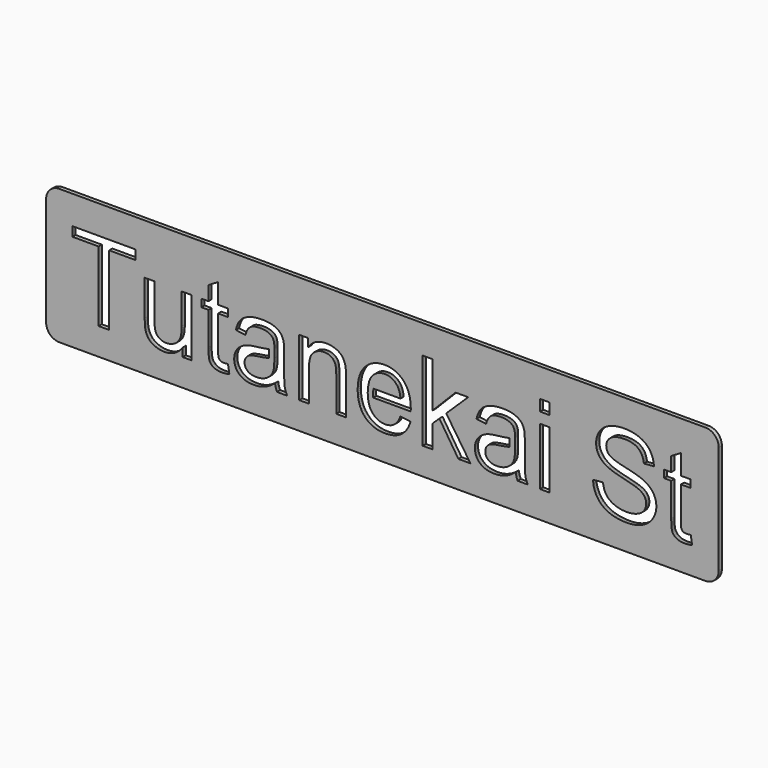
from build123d import *

# Parameters (mm, degrees)
F0_W     = 7.366985
F0_H     = 43.465212
F0_H_2   = 8.472032
F1_DEPTH = 3


# Not quite as in the source:
# - ends of sketch curves that miss each other by under 0.0002 mm in the source are joined


with BuildPart() as f1:
    # F0 (on Front) → F1 (new body)
    with BuildSketch(Plane.XZ):
        with BuildLine():
            Line((-254, 41), (-254, -41))
            ThreePointArc((-254, -41), (-251.0710678119, -48.0710678119), (-244, -51))
            Line((-244, -51), (244, -51))
            ThreePointArc((244, -51), (251.0710678119, -48.0710678119), (254, -41))
            Line((254, -41), (254, 41))
            ThreePointArc((254, 41), (251.0710678119, 48.0710678119), (244, 51))
            Line((244, 51), (-244, 51))
            ThreePointArc((-244, 51), (-251.0710678119, 48.0710678119), (-254, 41))
        make_face()
        Polygon((-206.388994, 22.359541), (-206.388994, -30.559968), (-214.328967, -30.559968), (-214.328967, 22.359541), (-234.097043, 22.359541), (-234.097043, 29.440032), (-186.539063, 29.440032), (-186.539063, 22.359541), align=None, mode=Mode.SUBTRACT)
        Polygon((-144.260754, 12.905244), (-144.260754, -30.559968), (-150.850113, -30.559968), (-150.850113, -24.175247), (-151.498721, -25.067343), (-152.175787, -25.901884), (-152.88131, -26.678871), (-153.61529, -27.398303), (-154.377729, -28.060181), (-155.168624, -28.664504), (-155.987977, -29.211272), (-156.835788, -29.700486), (-157.712057, -30.132145), (-158.616782, -30.50625), (-159.549966, -30.8228), (-160.511607, -31.081796), (-161.501705, -31.283237), (-162.520261, -31.427123), (-163.567275, -31.513455), (-164.642746, -31.542232), (-165.596553, -31.51921), (-166.534373, -31.450145), (-167.456205, -31.335036), (-168.36205, -31.173883), (-169.251908, -30.966686), (-170.125778, -30.713446), (-170.983661, -30.414163), (-171.825556, -30.068835), (-172.632599, -29.688655), (-173.385925, -29.284814), (-174.085532, -28.857311), (-174.731423, -28.406148), (-175.323595, -27.931322), (-175.86205, -27.432836), (-176.346788, -26.910688), (-176.777807, -26.364879), (-177.16694, -25.791571), (-177.526017, -25.186929), (-177.855037, -24.550951), (-178.154001, -23.883637), (-178.422909, -23.184989), (-178.66176, -22.455005), (-178.870556, -21.693686), (-179.049294, -20.901032), (-179.154811, -20.319091), (-179.246259, -19.657853), (-179.323638, -18.917317), (-179.386948, -18.097485), (-179.436189, -17.198354), (-179.471361, -16.219927), (-179.492465, -15.162201), (-179.499499, -14.025179), (-179.499499, 12.905244), (-172.132514, 12.905244), (-172.132514, -11.201168), (-172.130755, -11.90781), (-172.12548, -12.585036), (-172.116687, -13.232844), (-172.104376, -13.851236), (-172.088549, -14.440211), (-172.069204, -14.99977), (-172.046342, -15.529911), (-172.019963, -16.030636), (-171.990067, -16.501944), (-171.956653, -16.943835), (-171.919722, -17.35631), (-171.879274, -17.739367), (-171.835309, -18.093008), (-171.787826, -18.417232), (-171.736826, -18.712039), (-171.682309, -18.97743), (-171.484066, -19.684392), (-171.237221, -20.352345), (-170.941774, -20.981288), (-170.597726, -21.571223), (-170.205075, -22.122148), (-169.763824, -22.634064), (-169.27397, -23.10697), (-168.735515, -23.540868), (-168.156133, -23.929361), (-167.543496, -24.266056), (-166.897606, -24.550951), (-166.218462, -24.784047), (-165.506065, -24.965344), (-164.760413, -25.094841), (-163.981508, -25.17254), (-163.169349, -25.19844), (-162.346958, -25.171901), (-161.537357, -25.092283), (-160.740546, -24.959588), (-159.956525, -24.773815), (-159.185294, -24.534963), (-158.426852, -24.243034), (-157.681201, -23.898026), (-156.948339, -23.49994), (-156.248412, -23.056131), (-155.601563, -22.573951), (-155.007791, -22.053402), (-154.467098, -21.494483), (-153.979483, -20.897195), (-153.544946, -20.261536), (-153.163487, -19.587508), (-152.835106, -18.875111), (-152.55213, -18.102281), (-152.306883, -17.246956), (-152.099367, -16.309136), (-151.929581, -15.288822), (-151.797525, -14.186012), (-151.7032, -13.000708), (-151.646604, -11.732908), (-151.627739, -10.382614), (-151.627739, 12.905244), align=None, mode=Mode.SUBTRACT)
        Polygon((-97.552982, 7.077844), (-97.979446, 6.928442), (-98.384646, 6.764811), (-98.768583, 6.586951), (-99.131256, 6.394863), (-99.472667, 6.188546), (-99.792814, 5.968), (-100.097294, 5.729388), (-100.391701, 5.468874), (-100.676037, 5.186457), (-100.950301, 4.882137), (-101.214492, 4.555914), (-101.468611, 4.207789), (-101.712659, 3.837761), (-101.946634, 3.445831), (-102.170537, 3.031997), (-102.384369, 2.596261), (-102.588128, 2.138622), (-102.781815, 1.659081), (-102.96543, 1.157637), (-103.138973, 0.63429), (-103.302444, 0.08904), (-103.455843, -0.478112), (-110.659117, 0.504153), (-110.393727, 1.632542), (-110.088687, 2.705295), (-109.743999, 3.722412), (-109.359663, 4.683893), (-108.935677, 5.589738), (-108.472043, 6.439947), (-107.968761, 7.23452), (-107.425829, 7.973457), (-106.831738, 8.664112), (-106.174977, 9.313839), (-105.455544, 9.922638), (-104.673442, 10.49051), (-103.828669, 11.017454), (-102.921225, 11.50347), (-101.951111, 11.948559), (-100.918326, 12.35272), (-99.833102, 12.712436), (-98.705672, 13.02419), (-97.536036, 13.287982), (-96.324192, 13.503811), (-95.070142, 13.671679), (-93.773885, 13.791584), (-92.435422, 13.863528), (-91.054751, 13.887509), (-89.695824, 13.867045), (-88.402125, 13.805653), (-87.173655, 13.703334), (-86.010413, 13.560087), (-84.9124, 13.375912), (-83.879615, 13.15081), (-82.912059, 12.88478), (-82.009731, 12.577822), (-81.168795, 12.239849), (-80.385413, 11.880773), (-79.659586, 11.500593), (-78.991314, 11.099309), (-78.380596, 10.676923), (-77.827432, 10.233433), (-77.331823, 9.76884), (-76.893769, 9.283143), (-76.49984, 8.770588), (-76.136607, 8.225418), (-75.804069, 7.647634), (-75.502228, 7.037236), (-75.231082, 6.394223), (-74.990631, 5.718597), (-74.780877, 5.010356), (-74.601818, 4.2695), (-74.515486, 3.751509), (-74.440666, 3.138873), (-74.377355, 2.431591), (-74.325556, 1.629664), (-74.285268, 0.733092), (-74.256491, -0.258126), (-74.239225, -1.343989), (-74.233469, -2.524497), (-74.233469, -12.347144), (-74.231631, -13.601753), (-74.226115, -14.797369), (-74.216922, -15.933992), (-74.204052, -17.011622), (-74.187505, -18.030258), (-74.167281, -18.9899), (-74.14338, -19.890549), (-74.115802, -20.732205), (-74.084547, -21.514867), (-74.049614, -22.238536), (-74.011005, -22.903211), (-73.968718, -23.508893), (-73.922754, -24.055582), (-73.873113, -24.543277), (-73.819796, -24.971978), (-73.762801, -25.341686), (-73.630745, -26.018592), (-73.469912, -26.688463), (-73.280301, -27.3513), (-73.061914, -28.007103), (-72.814749, -28.65587), (-72.538807, -29.297604), (-72.234087, -29.932303), (-71.90059, -30.559968), (-79.594997, -30.559968), (-79.868701, -29.974829), (-80.116825, -29.36539), (-80.339369, -28.731651), (-80.536334, -28.07361), (-80.707719, -27.391269), (-80.853524, -26.684626), (-80.973749, -25.953683), (-81.068394, -25.19844), (-82.08679, -26.036178), (-83.095594, -26.809968), (-84.094805, -27.519807), (-85.084424, -28.165697), (-86.06445, -28.747638), (-87.034884, -29.265629), (-87.995726, -29.719671), (-88.946975, -30.109763), (-89.902061, -30.445498), (-90.874414, -30.736468), (-91.864033, -30.982674), (-92.870918, -31.184115), (-93.895069, -31.340791), (-94.936487, -31.452703), (-95.995172, -31.51985), (-97.071123, -31.542232), (-97.953466, -31.528563), (-98.80991, -31.487555), (-99.640454, -31.419209), (-100.445099, -31.323525), (-101.223845, -31.200502), (-101.97669, -31.050141), (-102.703637, -30.872441), (-103.404683, -30.667403), (-104.07983, -30.435026), (-104.729078, -30.175311), (-105.352426, -29.888258), (-105.949874, -29.573866), (-106.521423, -29.232136), (-107.067072, -28.863067), (-107.586822, -28.46666), (-108.080672, -28.042914), (-108.546545, -27.597906), (-108.982361, -27.137709), (-109.38812, -26.662324), (-109.763824, -26.171751), (-110.109471, -25.665991), (-110.425062, -25.145042), (-110.710596, -24.608905), (-110.966075, -24.05758), (-111.191497, -23.491067), (-111.386863, -22.909366), (-111.552172, -22.312478), (-111.687425, -21.700401), (-111.792622, -21.073136), (-111.867763, -20.430683), (-111.912847, -19.773042), (-111.927876, -19.100213), (-111.905174, -18.310756), (-111.837067, -17.538566), (-111.723557, -16.783642), (-111.564642, -16.045984), (-111.360324, -15.325593), (-111.110601, -14.622468), (-110.815474, -13.936609), (-110.474942, -13.268017), (-110.09764, -12.624365), (-109.6922, -12.013327), (-109.258623, -11.434904), (-108.796907, -10.889094), (-108.307054, -10.375899), (-107.789063, -9.895319), (-107.242934, -9.447352), (-106.668667, -9.032), (-106.071059, -8.645106), (-105.454905, -8.282512), (-104.820206, -7.944219), (-104.166962, -7.630227), (-103.495172, -7.340535), (-102.804837, -7.075145), (-102.095956, -6.834055), (-101.36853, -6.617266), (-100.791706, -6.474659), (-100.145816, -6.33333), (-99.43086, -6.193281), (-98.646839, -6.05451), (-97.793752, -5.917019), (-96.8716, -5.780807), (-95.880382, -5.645873), (-94.820099, -5.512219), (-93.723205, -5.377605), (-92.663082, -5.239794), (-91.63973, -5.098785), (-90.653148, -4.954579), (-89.703338, -4.807175), (-88.790299, -4.656574), (-87.914031, -4.502775), (-87.074533, -4.345779), (-86.271807, -4.185586), (-85.674982, -4.058273), (-85.684298, -10.013809), (-85.959573, -10.08397), (-86.695952, -10.259831), (-87.463666, -10.431855), (-88.262715, -10.600043), (-89.0931, -10.764393), (-89.95482, -10.924906), (-90.847875, -11.081582), (-91.772265, -11.234422), (-92.727991, -11.383424), (-93.715052, -11.52859), (-94.809228, -11.694858), (-95.82027, -11.866243), (-96.748177, -12.042744), (-97.592951, -12.22436), (-98.354589, -12.411093), (-99.033094, -12.602942), (-99.628464, -12.799906), (-100.1407, -13.001987), (-100.597939, -13.218456), (-101.028319, -13.458586), (-101.43184, -13.722378), (-101.808503, -14.009831), (-102.158307, -14.320946), (-102.481252, -14.655721), (-102.777338, -15.014158), (-103.046566, -15.396257), (-103.286377, -15.795622), (-103.494213, -16.205858), (-103.670074, -16.626965), (-103.81396, -17.058944), (-103.925872, -17.501795), (-104.005809, -17.955517), (-104.053771, -18.42011), (-104.069758, -18.895575), (-104.034906, -19.616925), (-103.930348, -20.30758), (-103.756086, -20.967539), (-103.512118, -21.596802), (-103.198446, -22.19537), (-102.815069, -22.763242), (-102.361986, -23.300418), (-101.839199, -23.806898), (-101.249265, -24.267335), (-100.594741, -24.66638), (-99.875629, -25.004033), (-99.091927, -25.280295), (-98.243637, -25.495165), (-97.330758, -25.648644), (-96.353289, -25.740732), (-95.311232, -25.771427), (-94.26182, -25.74233), (-93.241825, -25.655039), (-92.251247, -25.509554), (-91.290086, -25.305875), (-90.358341, -25.044001), (-89.456013, -24.723934), (-88.583102, -24.345673), (-87.739608, -23.909217), (-86.938321, -23.422242), (-86.19203, -22.89242), (-85.500735, -22.319752), (-84.864438, -21.704238), (-84.283137, -21.045877), (-83.756832, -20.344671), (-83.285524, -19.600618), (-82.869213, -18.813719), (-82.591032, -18.152481), (-82.349942, -17.417062), (-82.145943, -16.607461), (-81.979035, -15.723678), (-81.849218, -14.765714), (-81.756491, -13.733569), (-81.700855, -12.627242), (-81.682309, -11.446734), (-81.682309, -8.745506), (-81.672717, -2.613387), (-81.664404, -2.286605), (-81.657369, -1.994355), (-81.651614, -1.736639), (-81.647137, -1.513455), (-81.64394, -1.324804), (-81.642021, -1.170685), (-81.641382, -1.0511), (-81.649535, -0.498736), (-81.673996, 0.032845), (-81.714764, 0.543641), (-81.771839, 1.033655), (-81.845221, 1.502884), (-81.93491, 1.95133), (-82.040906, 2.378993), (-82.16321, 2.785871), (-82.30182, 3.171967), (-82.456738, 3.537278), (-82.627963, 3.881806), (-82.815495, 4.205551), (-83.019334, 4.508512), (-83.23948, 4.790689), (-83.475934, 5.052083), (-83.728694, 5.292693), (-84.092407, 5.595014), (-84.477543, 5.877831), (-84.884102, 6.141143), (-85.312084, 6.384951), (-85.76149, 6.609254), (-86.232318, 6.814052), (-86.724569, 6.999346), (-87.238244, 7.165135), (-87.773342, 7.311419), (-88.329862, 7.438199), (-88.907806, 7.545475), (-89.507173, 7.633245), (-90.127963, 7.701511), (-90.770176, 7.750273), (-91.433812, 7.77953), (-92.118872, 7.789282), (-92.757967, 7.782168), (-93.375799, 7.760825), (-93.972368, 7.725253), (-94.547674, 7.675452), (-95.101717, 7.611423), (-95.634497, 7.533164), (-96.146013, 7.440677), (-96.636266, 7.333962), (-97.105256, 7.213017), align=None, mode=Mode.SUBTRACT)
        Polygon((-117.588687, -24.09595), (-117.123774, -24.037756), (-116.63456, -23.970609), (-115.57044, -30.478112), (-116.337835, -30.631591), (-117.084765, -30.764606), (-117.811232, -30.877157), (-118.517234, -30.969244), (-119.202773, -31.040868), (-119.867848, -31.092028), (-120.51246, -31.122723), (-121.136607, -31.132955), (-122.111198, -31.113131), (-123.029513, -31.053658), (-123.891552, -30.954536), (-124.697316, -30.815766), (-125.446805, -30.637346), (-126.140017, -30.419279), (-126.776955, -30.161562), (-127.357616, -29.864197), (-127.889676, -29.534537), (-128.380809, -29.179937), (-128.831013, -28.800396), (-129.24029, -28.395916), (-129.60864, -27.966495), (-129.936061, -27.512133), (-130.222555, -27.032832), (-130.468121, -26.52859), (-130.577155, -26.252408), (-130.679155, -25.940574), (-130.77412, -25.593088), (-130.86205, -25.20995), (-130.942946, -24.791161), (-131.016808, -24.33672), (-131.083635, -23.846627), (-131.143428, -23.320882), (-131.196186, -22.759485), (-131.24191, -22.162436), (-131.2806, -21.529735), (-131.312255, -20.861383), (-131.336875, -20.157379), (-131.354462, -19.417722), (-131.365013, -18.642414), (-131.36853, -17.831455), (-131.36853, 7.175367), (-136.770986, 7.175367), (-136.770986, 12.905244), (-131.36853, 12.905244), (-131.36853, 23.669228), (-124.042473, 28.089419), (-124.042473, 12.905244), (-116.63456, 12.905244), (-116.63456, 7.175367), (-124.042473, 7.175367), (-124.042473, -18.240732), (-124.036398, -18.993417), (-124.018172, -19.675759), (-123.987796, -20.287756), (-123.94527, -20.829408), (-123.890593, -21.300716), (-123.823766, -21.70168), (-123.744788, -22.032299), (-123.65366, -22.292573), (-123.428558, -22.719756), (-123.142064, -23.100895), (-122.794178, -23.435991), (-122.384902, -23.725043), (-122.153085, -23.849744), (-121.897606, -23.957819), (-121.618466, -24.049267), (-121.315666, -24.124088), (-120.989203, -24.182282), (-120.63908, -24.223849), (-120.265295, -24.248789), (-119.867848, -24.257103), (-119.54874, -24.252626), (-119.205331, -24.239197), (-118.837622, -24.216814), (-118.445611, -24.185479), (-118.0293, -24.145191), align=None, mode=Mode.SUBTRACT)
        Polygon((-55.447657, -6.821905), (-55.447657, -30.559968), (-62.814642, -30.559968), (-62.814642, 12.905244), (-56.184356, 12.905244), (-56.184356, 6.725162), (-55.569161, 7.592477), (-54.920713, 8.403837), (-54.239011, 9.159241), (-53.524056, 9.858689), (-52.775846, 10.502181), (-51.994383, 11.089717), (-51.179666, 11.621297), (-50.331696, 12.096922), (-49.450471, 12.516591), (-48.535993, 12.880304), (-47.588261, 13.188061), (-46.607275, 13.439862), (-45.593036, 13.635707), (-44.545543, 13.775597), (-43.464796, 13.859531), (-42.350795, 13.887509), (-41.378443, 13.865446), (-40.425914, 13.799258), (-39.493211, 13.688945), (-38.580331, 13.534507), (-37.687276, 13.335944), (-36.814045, 13.093256), (-35.960639, 12.806442), (-35.127057, 12.475503), (-34.329287, 12.108753), (-33.583316, 11.714504), (-32.889144, 11.292757), (-32.246771, 10.843511), (-31.656197, 10.366768), (-31.117422, 9.862526), (-30.630446, 9.330785), (-30.19527, 8.771547), (-29.801341, 8.18513), (-29.438108, 7.571854), (-29.10557, 6.931719), (-28.803728, 6.264726), (-28.532582, 5.570873), (-28.292132, 4.850162), (-28.082378, 4.102592), (-27.903319, 3.328163), (-27.853758, 3.060375), (-27.807395, 2.768605), (-27.764229, 2.452854), (-27.72426, 2.113123), (-27.687489, 1.74941), (-27.653916, 1.361716), (-27.62354, 0.950041), (-27.596361, 0.514384), (-27.57238, 0.054747), (-27.551597, -0.428871), (-27.53401, -0.93647), (-27.519622, -1.468051), (-27.508431, -2.023612), (-27.500437, -2.603155), (-27.495641, -3.206678), (-27.494042, -3.834183), (-27.494042, -30.559968), (-34.861027, -30.559968), (-34.861027, -4.120677), (-34.874456, -3.030657), (-34.914745, -2.011622), (-34.981892, -1.06357), (-35.075897, -0.186502), (-35.196762, 0.619581), (-35.344485, 1.354681), (-35.519068, 2.018797), (-35.720509, 2.611929), (-35.956163, 3.1555), (-36.233384, 3.670933), (-36.552172, 4.158228), (-36.912528, 4.617386), (-37.31445, 5.048406), (-37.75794, 5.451288), (-38.242998, 5.826032), (-38.769622, 6.172638), (-39.32886, 6.484392), (-39.91176, 6.754579), (-40.518322, 6.983198), (-41.148544, 7.170251), (-41.802428, 7.315736), (-42.479973, 7.419654), (-43.18118, 7.482005), (-43.906047, 7.502788), (-44.489347, 7.491117), (-45.062575, 7.456105), (-45.62573, 7.397751), (-46.178814, 7.316056), (-46.721825, 7.211019), (-47.254764, 7.08264), (-47.777632, 6.93092), (-48.290427, 6.755858), (-48.79315, 6.557454), (-49.285801, 6.335709), (-49.76838, 6.090623), (-50.240887, 5.822195), (-50.703322, 5.530425), (-51.155685, 5.215314), (-51.597976, 4.876861), (-52.030195, 4.515067), (-52.444028, 4.120658), (-52.831163, 3.684362), (-53.191598, 3.20618), (-53.525335, 2.68611), (-53.832372, 2.124154), (-54.112711, 1.52031), (-54.366351, 0.87458), (-54.593292, 0.186963), (-54.793534, -0.542541), (-54.967077, -1.313932), (-55.113921, -2.12721), (-55.234066, -2.982375), (-55.327512, -3.879427), (-55.394259, -4.818366), (-55.434308, -5.799192), align=None, mode=Mode.SUBTRACT)
        with BuildLine():
            Line((-5.055434, -23.343903), (-4.536803, -23.685873))
            Line((-4.536803, -23.685873), (-4.004103, -23.998107))
            Line((-4.004103, -23.998107), (-3.457335, -24.280604))
            Line((-3.457335, -24.280604), (-2.896498, -24.533365))
            Line((-2.896498, -24.533365), (-2.321591, -24.756388))
            Line((-2.321591, -24.756388), (-1.732616, -24.949676))
            Line((-1.732616, -24.949676), (-1.129572, -25.113227))
            Line((-1.129572, -25.113227), (-0.51246, -25.247041))
            Line((-0.51246, -25.247041), (0.118722, -25.351119))
            Line((0.118722, -25.351119), (0.763973, -25.42546))
            Line((0.763973, -25.42546), (1.423293, -25.470065))
            Line((1.423293, -25.470065), (2.096681, -25.484933))
            Line((2.096681, -25.484933), (3.091096, -25.45168))
            Line((3.091096, -25.45168), (4.04842, -25.351918))
            Line((4.04842, -25.351918), (4.968654, -25.18565))
            Line((4.968654, -25.18565), (5.851797, -24.952873))
            Line((5.851797, -24.952873), (6.697849, -24.65359))
            Line((6.697849, -24.65359), (7.506811, -24.287798))
            Line((7.506811, -24.287798), (8.278681, -23.8555))
            Line((8.278681, -23.8555), (9.013461, -23.356693))
            Line((9.013461, -23.356693), (9.711151, -22.784985))
            Line((9.711151, -22.784985), (10.371749, -22.133978))
            Line((10.371749, -22.133978), (10.995257, -21.403675))
            Line((10.995257, -21.403675), (11.581674, -20.594074))
            Line((11.581674, -20.594074), (12.131001, -19.705176))
            Line((12.131001, -19.705176), (12.643236, -18.73698))
            Line((12.643236, -18.73698), (13.118381, -17.689487))
            Line((13.118381, -17.689487), (13.556435, -16.562696))
            Line((13.556435, -16.562696), (21.168987, -17.504033))
            Line((21.168987, -17.504033), (20.931894, -18.326264))
            Line((20.931894, -18.326264), (20.67082, -19.125153))
            Line((20.67082, -19.125153), (20.385765, -19.900701))
            Line((20.385765, -19.900701), (20.076729, -20.652907))
            Line((20.076729, -20.652907), (19.743712, -21.381772))
            Line((19.743712, -21.381772), (19.386713, -22.087295))
            Line((19.386713, -22.087295), (19.005734, -22.769477))
            Line((19.005734, -22.769477), (18.600774, -23.428317))
            Line((18.600774, -23.428317), (18.171832, -24.063815))
            Line((18.171832, -24.063815), (17.71891, -24.675972))
            Line((17.71891, -24.675972), (17.242006, -25.264787))
            Line((17.242006, -25.264787), (16.741122, -25.830261))
            Line((16.741122, -25.830261), (16.216256, -26.372393))
            Line((16.216256, -26.372393), (15.667409, -26.891183))
            Line((15.667409, -26.891183), (15.094581, -27.386632))
            Line((15.094581, -27.386632), (14.497772, -27.85874))
            Line((14.497772, -27.85874), (13.878421, -28.304788))
            Line((13.878421, -28.304788), (13.237967, -28.722058))
            Line((13.237967, -28.722058), (12.576409, -29.110552))
            Line((12.576409, -29.110552), (11.893748, -29.470268))
            Line((11.893748, -29.470268), (11.189983, -29.801206))
            Line((11.189983, -29.801206), (10.465116, -30.103368))
            Line((10.465116, -30.103368), (9.719144, -30.376752))
            Line((9.719144, -30.376752), (8.95207, -30.621359))
            Line((8.95207, -30.621359), (8.163892, -30.837189))
            Line((8.163892, -30.837189), (7.354611, -31.024241))
            Line((7.354611, -31.024241), (6.524226, -31.182516))
            Line((6.524226, -31.182516), (5.672738, -31.312014))
            Line((5.672738, -31.312014), (4.800147, -31.412734))
            Line((4.800147, -31.412734), (3.906453, -31.484678))
            Line((3.906453, -31.484678), (2.991655, -31.527844))
            Line((2.991655, -31.527844), (2.055753, -31.542232))
            Line((2.055753, -31.542232), (0.879162, -31.51929))
            Line((0.879162, -31.51929), (-0.266574, -31.450465))
            Line((-0.266574, -31.450465), (-1.381454, -31.335755))
            Line((-1.381454, -31.335755), (-2.465478, -31.175162))
            Line((-2.465478, -31.175162), (-3.518647, -30.968685))
            Line((-3.518647, -30.968685), (-4.54096, -30.716324))
            Line((-4.54096, -30.716324), (-5.532417, -30.41808))
            Line((-5.532417, -30.41808), (-6.493019, -30.073951))
            Line((-6.493019, -30.073951), (-7.422765, -29.683939))
            Line((-7.422765, -29.683939), (-8.321655, -29.248043))
            Line((-8.321655, -29.248043), (-9.18969, -28.766263))
            Line((-9.18969, -28.766263), (-10.026869, -28.2386))
            Line((-10.026869, -28.2386), (-10.833193, -27.665053))
            Line((-10.833193, -27.665053), (-11.608661, -27.045622))
            Line((-11.608661, -27.045622), (-12.353273, -26.380307))
            Line((-12.353273, -26.380307), (-13.06703, -25.669108))
            Line((-13.06703, -25.669108), (-13.743536, -24.916502))
            Line((-13.743536, -24.916502), (-14.376396, -24.126965))
            Line((-14.376396, -24.126965), (-14.965611, -23.300498))
            Line((-14.965611, -23.300498), (-15.511181, -22.437099))
            Line((-15.511181, -22.437099), (-16.013104, -21.53677))
            Line((-16.013104, -21.53677), (-16.471383, -20.59951))
            Line((-16.471383, -20.59951), (-16.886015, -19.625319))
            Line((-16.886015, -19.625319), (-17.257002, -18.614197))
            Line((-17.257002, -18.614197), (-17.584344, -17.566144))
            Line((-17.584344, -17.566144), (-17.86804, -16.48116))
            Line((-17.86804, -16.48116), (-18.108091, -15.359246))
            Line((-18.108091, -15.359246), (-18.304496, -14.200401))
            Line((-18.304496, -14.200401), (-18.457255, -13.004625))
            Line((-18.457255, -13.004625), (-18.566369, -11.771918))
            Line((-18.566369, -11.771918), (-18.631837, -10.50228))
            Line((-18.631837, -10.50228), (-18.65366, -9.195711))
            Line((-18.65366, -9.195711), (-18.631597, -7.843818))
            Line((-18.631597, -7.843818), (-18.56541, -6.530295))
            Line((-18.56541, -6.530295), (-18.455097, -5.255141))
            Line((-18.455097, -5.255141), (-18.300659, -4.018358))
            Line((-18.300659, -4.018358), (-18.102095, -2.819944))
            Line((-18.102095, -2.819944), (-17.859407, -1.659899))
            Line((-17.859407, -1.659899), (-17.572593, -0.538225))
            Line((-17.572593, -0.538225), (-17.241655, 0.54508))
            Line((-17.241655, 0.54508), (-16.866591, 1.590015))
            Line((-16.866591, 1.590015), (-16.447402, 2.596581))
            Line((-16.447402, 2.596581), (-15.984087, 3.564777))
            Line((-15.984087, 3.564777), (-15.476648, 4.494603))
            Line((-15.476648, 4.494603), (-14.925083, 5.386059))
            Line((-14.925083, 5.386059), (-14.329393, 6.239146))
            Line((-14.329393, 6.239146), (-13.689578, 7.053863))
            Line((-13.689578, 7.053863), (-13.005638, 7.83021))
            Line((-13.005638, 7.83021), (-12.286526, 8.563711))
            Line((-12.286526, 8.563711), (-11.541194, 9.249889))
            Line((-11.541194, 9.249889), (-10.769643, 9.888745))
            Line((-10.769643, 9.888745), (-9.971873, 10.480278))
            Line((-9.971873, 10.480278), (-9.147883, 11.024488))
            Line((-9.147883, 11.024488), (-8.297674, 11.521376))
            Line((-8.297674, 11.521376), (-7.421246, 11.970941))
            Line((-7.421246, 11.970941), (-6.518599, 12.373184))
            Line((-6.518599, 12.373184), (-5.589732, 12.728104))
            Line((-5.589732, 12.728104), (-4.634646, 13.035701))
            Line((-4.634646, 13.035701), (-3.65334, 13.295976))
            Line((-3.65334, 13.295976), (-2.645816, 13.508927))
            Line((-2.645816, 13.508927), (-1.612072, 13.674557))
            Line((-1.612072, 13.674557), (-0.552108, 13.792863))
            Line((-0.552108, 13.792863), (0.534074, 13.863847))
            Line((0.534074, 13.863847), (1.646476, 13.887509))
            Line((1.646476, 13.887509), (2.723706, 13.864327))
            Line((2.723706, 13.864327), (3.775995, 13.794782))
            Line((3.775995, 13.794782), (4.803345, 13.678873))
            Line((4.803345, 13.678873), (5.805753, 13.516601))
            Line((5.805753, 13.516601), (6.783222, 13.307966))
            Line((6.783222, 13.307966), (7.73575, 13.052967))
            Line((7.73575, 13.052967), (8.663338, 12.751605))
            Line((8.663338, 12.751605), (9.565985, 12.40388))
            Line((9.565985, 12.40388), (10.443692, 12.009791))
            Line((10.443692, 12.009791), (11.296459, 11.569338))
            Line((11.296459, 11.569338), (12.124286, 11.082523))
            Line((12.124286, 11.082523), (12.927172, 10.549344))
            Line((12.927172, 10.549344), (13.705118, 9.969801))
            Line((13.705118, 9.969801), (14.458124, 9.343895))
            Line((14.458124, 9.343895), (15.186189, 8.671626))
            Line((15.186189, 8.671626), (15.889314, 7.952993))
            Line((15.889314, 7.952993), (16.558386, 7.192313))
            Line((16.558386, 7.192313), (17.184292, 6.393904))
            Line((17.184292, 6.393904), (17.767032, 5.557764))
            Line((17.767032, 5.557764), (18.306606, 4.683893))
            Line((18.306606, 4.683893), (18.803014, 3.772293))
            Line((18.803014, 3.772293), (19.256256, 2.822962))
            Line((19.256256, 2.822962), (19.666333, 1.835901))
            Line((19.666333, 1.835901), (20.033243, 0.81111))
            Line((20.033243, 0.81111), (20.356988, -0.251411))
            Line((20.356988, -0.251411), (20.637566, -1.351663))
            Line((20.637566, -1.351663), (20.874979, -2.489644))
            Line((20.874979, -2.489644), (21.069225, -3.665356))
            Line((21.069225, -3.665356), (21.220306, -4.878799))
            Line((21.220306, -4.878799), (21.328221, -6.129971))
            Line((21.328221, -6.129971), (21.39297, -7.418874))
            Line((21.39297, -7.418874), (21.414553, -8.745506))
            Line((21.414553, -8.745506), (21.411995, -9.113856))
            Line((21.411995, -9.113856), (21.404321, -9.56406))
            Line((21.404321, -9.56406), (21.391531, -10.09612))
            Line((21.391531, -10.09612), (21.373625, -10.710036))
            Line((21.373625, -10.710036), (-7.030793, -10.710036))
            ThreePointArc((-7.030793, -10.710036), (-7.0759469375, -7.672327893), (-6.7416103188, -4.6527371189))
            Line((-6.7416103188, -4.6527371189), (13.638291, -4.652737))
            Line((13.638291, -4.652737), (13.569865, -3.97791))
            Line((13.569865, -3.97791), (13.48737, -3.324505))
            Line((13.48737, -3.324505), (13.390806, -2.692524))
            Line((13.390806, -2.692524), (13.280174, -2.081966))
            Line((13.280174, -2.081966), (13.155472, -1.492831))
            Line((13.155472, -1.492831), (13.016701, -0.925119))
            Line((13.016701, -0.925119), (12.863862, -0.37883))
            Line((12.863862, -0.37883), (12.696954, 0.146035))
            Line((12.696954, 0.146035), (12.515977, 0.649478))
            Line((12.515977, 0.649478), (12.320931, 1.131497))
            Line((12.320931, 1.131497), (12.111816, 1.592094))
            Line((12.111816, 1.592094), (11.888632, 2.031267))
            Line((11.888632, 2.031267), (11.651379, 2.449017))
            Line((11.651379, 2.449017), (11.400058, 2.845345))
            Line((11.400058, 2.845345), (11.134667, 3.220249))
            Line((11.134667, 3.220249), (10.855208, 3.57373))
            Line((10.855208, 3.57373), (10.407081, 4.089163))
            Line((10.407081, 4.089163), (9.942648, 4.571342))
            Line((9.942648, 4.571342), (9.461907, 5.020268))
            Line((9.461907, 5.020268), (8.96486, 5.43594))
            Line((8.96486, 5.43594), (8.451505, 5.818358))
            Line((8.451505, 5.818358), (7.921843, 6.167522))
            Line((7.921843, 6.167522), (7.375874, 6.483433))
            Line((7.375874, 6.483433), (6.813598, 6.76609))
            Line((6.813598, 6.76609), (6.235014, 7.015493))
            Line((6.235014, 7.015493), (5.640124, 7.231642))
            Line((5.640124, 7.231642), (5.028926, 7.414538))
            Line((5.028926, 7.414538), (4.401422, 7.56418))
            Line((4.401422, 7.56418), (3.75761, 7.680568))
            Line((3.75761, 7.680568), (3.097491, 7.763702))
            Line((3.097491, 7.763702), (2.421065, 7.813583))
            Line((2.421065, 7.813583), (1.728332, 7.83021))
            Line((1.728332, 7.83021), (1.100268, 7.81694))
            Line((1.100268, 7.81694), (0.484833, 7.777132))
            Line((0.484833, 7.777132), (-0.117971, 7.710784))
            Line((-0.117971, 7.710784), (-0.708145, 7.617897))
            Line((-0.708145, 7.617897), (-1.285689, 7.498472))
            Line((-1.285689, 7.498472), (-1.850603, 7.352507))
            Line((-1.850603, 7.352507), (-2.402887, 7.180003))
            Line((-2.402887, 7.180003), (-2.942541, 6.98096))
            Line((-2.942541, 6.98096), (-3.469565, 6.755378))
            Line((-3.469565, 6.755378), (-3.983959, 6.503257))
            Line((-3.983959, 6.503257), (-4.485723, 6.224597))
            Line((-4.485723, 6.224597), (-4.974857, 5.919398))
            Line((-4.974857, 5.919398), (-5.451361, 5.58766))
            Line((-5.451361, 5.58766), (-5.915235, 5.229383))
            Line((-5.915235, 5.229383), (-6.366479, 4.844566))
            Line((-6.366479, 4.844566), (-6.805093, 4.433211))
            Line((-6.805093, 4.433211), (-7.225321, 3.999633))
            Line((-7.225321, 3.999633), (-7.621408, 3.54815))
            Line((-7.621408, 3.54815), (-7.993355, 3.07876))
            Line((-7.993355, 3.07876), (-8.34116, 2.591465))
            Line((-8.34116, 2.591465), (-8.664825, 2.086264))
            Line((-8.664825, 2.086264), (-8.964348, 1.563157))
            Line((-8.964348, 1.563157), (-9.239731, 1.022144))
            Line((-9.239731, 1.022144), (-9.490972, 0.463225))
            Line((-9.490972, 0.463225), (-9.718073, -0.1136))
            Line((-9.718073, -0.1136), (-9.921033, -0.70833))
            Line((-9.921033, -0.70833), (-10.099852, -1.320967))
            Line((-10.099852, -1.320967), (-10.25453, -1.951509))
            ThreePointArc((-10.25453, -1.951509), (-11.1035378291, -8.7791510241), (-10.2794698989, -15.6098479751))
            Line((-10.2794698989, -15.6098479751), (-9.82351, -17.033365))
            Line((-9.82351, -17.033365), (-9.55764, -17.705794))
            Line((-9.55764, -17.705794), (-9.26651, -18.352004))
            Line((-9.26651, -18.352004), (-8.950119, -18.971994))
            Line((-8.950119, -18.971994), (-8.608469, -19.565766))
            Line((-8.608469, -19.565766), (-8.241559, -20.133318))
            Line((-8.241559, -20.133318), (-7.849388, -20.67465))
            Line((-7.849388, -20.67465), (-7.431958, -21.189764))
            Line((-7.431958, -21.189764), (-6.989267, -21.678658))
            Line((-6.989267, -21.678658), (-6.526912, -22.139574))
            Line((-6.526912, -22.139574), (-6.050488, -22.570754))
            Line((-6.050488, -22.570754), (-5.559995, -22.972197))
            Line((-5.559995, -22.972197), (-5.055434, -23.343903))
        make_face(mode=Mode.SUBTRACT)
        Polygon((37.826558, -13.329408), (37.826558, -30.559968), (30.459573, -30.559968), (30.459573, 29.440032), (37.826558, 29.440032), (37.826558, -4.77552), (55.261756, 12.905244), (64.797909, 12.905244), (48.181265, -3.220268), (66.475944, -30.559968), (57.389996, -30.559968), (43.024375, -8.336229), align=None, mode=Mode.SUBTRACT)
        Polygon((90.326079, 7.77953), (89.641019, 7.789282), (89.001924, 7.782168), (88.384091, 7.760825), (87.787522, 7.725253), (87.212216, 7.675452), (86.658174, 7.611423), (86.125394, 7.533164), (85.613878, 7.440677), (85.123625, 7.333962), (84.654635, 7.213017), (84.206909, 7.077844), (83.780445, 6.928442), (83.375245, 6.764811), (82.991308, 6.586951), (82.628634, 6.394863), (82.287224, 6.188546), (81.967077, 5.968), (81.662597, 5.729388), (81.368189, 5.468874), (81.083854, 5.186457), (80.80959, 4.882137), (80.545399, 4.555914), (80.291279, 4.207789), (80.047232, 3.837761), (79.813257, 3.445831), (79.589353, 3.031997), (79.375522, 2.596261), (79.171763, 2.138622), (78.978076, 1.659081), (78.794461, 1.157637), (78.620918, 0.63429), (78.457447, 0.08904), (78.304048, -0.478112), (71.100774, 0.504153), (71.366164, 1.632542), (71.671204, 2.705295), (72.015891, 3.722412), (72.400228, 4.683893), (72.824213, 5.589738), (73.287847, 6.439947), (73.79113, 7.23452), (74.334062, 7.973457), (74.928153, 8.664112), (75.584914, 9.313839), (76.304346, 9.922638), (77.086449, 10.49051), (77.931222, 11.017454), (78.838666, 11.50347), (79.80878, 11.948559), (80.841565, 12.35272), (81.926788, 12.712436), (83.054219, 13.02419), (84.223855, 13.287982), (85.435699, 13.503811), (86.689749, 13.671679), (87.986006, 13.791584), (89.324469, 13.863528), (90.705139, 13.887509), (92.064067, 13.867045), (93.357766, 13.805653), (94.586236, 13.703334), (95.749478, 13.560087), (96.847491, 13.375912), (97.880276, 13.15081), (98.847832, 12.88478), (99.75016, 12.577822), (100.591096, 12.239849), (101.374478, 11.880773), (102.100305, 11.500593), (102.768577, 11.099309), (103.379295, 10.676923), (103.932459, 10.233433), (104.428067, 9.76884), (104.866122, 9.283143), (105.260051, 8.770588), (105.623284, 8.225418), (105.955822, 7.647634), (106.257663, 7.037236), (106.528809, 6.394223), (106.769259, 5.718597), (106.979014, 5.010356), (107.158073, 4.2695), (107.244404, 3.751509), (107.319225, 3.138873), (107.382535, 2.431591), (107.434334, 1.629664), (107.474623, 0.733092), (107.5034, -0.258126), (107.520666, -1.343989), (107.526422, -2.524497), (107.526422, -12.347144), (107.52826, -13.601753), (107.533776, -14.797369), (107.542969, -15.933992), (107.555839, -17.011622), (107.572386, -18.030258), (107.59261, -18.9899), (107.616511, -19.890549), (107.644089, -20.732205), (107.675344, -21.514867), (107.710277, -22.238536), (107.748886, -22.903211), (107.791173, -23.508893), (107.837137, -24.055582), (107.886777, -24.543277), (107.940095, -24.971978), (107.99709, -25.341686), (108.129146, -26.018592), (108.289979, -26.688463), (108.479589, -27.3513), (108.697977, -28.007103), (108.945142, -28.65587), (109.221084, -29.297604), (109.525804, -29.932303), (109.8593, -30.559968), (102.164894, -30.559968), (101.89119, -29.974829), (101.643066, -29.36539), (101.420521, -28.731651), (101.223557, -28.07361), (101.052172, -27.391269), (100.906367, -26.684626), (100.786142, -25.953683), (100.691497, -25.19844), (99.673101, -26.036178), (98.664297, -26.809968), (97.665086, -27.519807), (96.675467, -28.165697), (95.69544, -28.747638), (94.725006, -29.265629), (93.764165, -29.719671), (92.812916, -30.109763), (91.85783, -30.445498), (90.885477, -30.736468), (89.895858, -30.982674), (88.888973, -31.184115), (87.864821, -31.340791), (86.823403, -31.452703), (85.764719, -31.51985), (84.688768, -31.542232), (83.806425, -31.528563), (82.949981, -31.487555), (82.119436, -31.419209), (81.314792, -31.323525), (80.536046, -31.200502), (79.7832, -31.050141), (79.056254, -30.872441), (78.355208, -30.667403), (77.680061, -30.435026), (77.030813, -30.175311), (76.407465, -29.888258), (75.810017, -29.573866), (75.238468, -29.232136), (74.692818, -28.863067), (74.173069, -28.46666), (73.679219, -28.042914), (73.213346, -27.597906), (72.77753, -27.137709), (72.371771, -26.662324), (71.996067, -26.171751), (71.65042, -25.665991), (71.334829, -25.145042), (71.049294, -24.608905), (70.793816, -24.05758), (70.568394, -23.491067), (70.373028, -22.909366), (70.207719, -22.312478), (70.072465, -21.700401), (69.967268, -21.073136), (69.892128, -20.430683), (69.847043, -19.773042), (69.832015, -19.100213), (69.854717, -18.310756), (69.922824, -17.538566), (70.036334, -16.783642), (70.195249, -16.045984), (70.399567, -15.325593), (70.64929, -14.622468), (70.944417, -13.936609), (71.284948, -13.268017), (71.662251, -12.624365), (72.067691, -12.013327), (72.501268, -11.434904), (72.962984, -10.889094), (73.452837, -10.375899), (73.970828, -9.895319), (74.516957, -9.447352), (75.091224, -9.032), (75.688832, -8.645106), (76.304986, -8.282512), (76.939685, -7.944219), (77.592929, -7.630227), (78.264719, -7.340535), (78.955054, -7.075145), (79.663935, -6.834055), (80.39136, -6.617266), (80.968185, -6.474659), (81.614075, -6.33333), (82.329031, -6.193281), (83.113052, -6.05451), (83.966139, -5.917019), (84.888291, -5.780807), (85.879508, -5.645873), (86.939792, -5.512219), (88.036686, -5.377605), (89.096809, -5.239794), (90.120161, -5.098785), (91.106742, -4.954579), (92.056553, -4.807175), (92.969592, -4.656574), (93.84586, -4.502775), (94.685358, -4.345779), (95.488084, -4.185586), (96.085603, -4.058125), (96.079136, -10.012906), (95.800318, -10.08397), (95.063939, -10.259831), (94.296225, -10.431855), (93.497176, -10.600043), (92.666791, -10.764393), (91.805071, -10.924906), (90.912016, -11.081582), (89.987626, -11.234422), (89.0319, -11.383424), (88.044839, -11.52859), (86.950663, -11.694858), (85.939621, -11.866243), (85.011713, -12.042744), (84.16694, -12.22436), (83.405301, -12.411093), (82.726797, -12.602942), (82.131427, -12.799906), (81.619191, -13.001987), (81.161952, -13.218456), (80.731572, -13.458586), (80.32805, -13.722378), (79.951388, -14.009831), (79.601584, -14.320946), (79.278639, -14.655721), (78.982552, -15.014158), (78.713325, -15.396257), (78.473514, -15.795622), (78.265678, -16.205858), (78.089817, -16.626965), (77.945931, -17.058944), (77.834019, -17.501795), (77.754082, -17.955517), (77.70612, -18.42011), (77.690133, -18.895575), (77.724985, -19.616925), (77.829543, -20.30758), (78.003805, -20.967539), (78.247772, -21.596802), (78.561445, -22.19537), (78.944822, -22.763242), (79.397905, -23.300418), (79.920692, -23.806898), (80.510626, -24.267335), (81.16515, -24.66638), (81.884262, -25.004033), (82.667963, -25.280295), (83.516254, -25.495165), (84.429133, -25.648644), (85.406602, -25.740732), (86.448659, -25.771427), (87.498071, -25.74233), (88.518066, -25.655039), (89.508644, -25.509554), (90.469805, -25.305875), (91.40155, -25.044001), (92.303877, -24.723934), (93.176788, -24.345673), (94.020283, -23.909217), (94.82157, -23.422242), (95.567861, -22.89242), (96.259155, -22.319752), (96.895453, -21.704238), (97.476754, -21.045877), (98.003059, -20.344671), (98.474367, -19.600618), (98.890678, -18.813719), (99.168859, -18.152481), (99.409948, -17.417062), (99.613947, -16.607461), (99.780856, -15.723678), (99.910673, -14.765714), (100.0034, -13.733569), (100.059036, -12.627242), (100.077581, -11.446734), (100.087174, -2.613387), (100.095487, -2.286605), (100.102522, -1.994355), (100.108277, -1.736639), (100.112754, -1.513455), (100.115951, -1.324804), (100.11787, -1.170685), (100.118509, -1.0511), (100.110356, -0.498736), (100.085895, 0.032845), (100.045127, 0.543641), (99.988052, 1.033655), (99.91467, 1.502884), (99.824981, 1.95133), (99.718984, 2.378993), (99.596681, 2.785871), (99.45807, 3.171967), (99.303153, 3.537278), (99.131928, 3.881806), (98.944396, 4.205551), (98.740557, 4.508512), (98.520411, 4.790689), (98.283957, 5.052083), (98.031197, 5.292693), (97.667484, 5.595014), (97.282348, 5.877831), (96.875789, 6.141143), (96.447807, 6.384951), (95.998401, 6.609254), (95.527573, 6.814052), (95.035321, 6.999346), (94.521647, 7.165135), (93.986549, 7.311419), (93.430029, 7.438199), (92.852085, 7.545475), (92.252718, 7.633245), (91.631928, 7.701511), (90.989715, 7.750273), align=None, mode=Mode.SUBTRACT)
        with Locations((122.6696685, -8.827362)):
            Rectangle(F0_W, F0_H, mode=Mode.SUBTRACT)
        Polygon((159.182608, -12.767612), (159.127371, -12.030194), (159.095317, -11.283023), (166.585085, -10.62818), (166.740162, -11.728432), (166.939365, -12.778163), (167.182693, -13.777375), (167.470146, -14.726066), (167.801724, -15.624237), (168.177428, -16.471888), (168.597257, -17.269019), (169.06121, -18.015629), (169.5808, -18.719713), (170.167537, -19.389265), (170.821421, -20.024284), (171.542452, -20.62477), (172.33063, -21.190723), (173.185955, -21.722144), (174.108426, -22.219031), (175.098045, -22.681386), (176.137225, -23.098657), (177.20838, -23.460292), (178.311509, -23.76629), (179.446613, -24.016652), (180.613692, -24.211379), (181.812745, -24.350469), (183.043773, -24.433923), (184.306777, -24.461741), (185.425893, -24.440638), (186.511756, -24.377328), (187.564365, -24.271811), (188.583721, -24.124088), (189.569822, -23.934157), (190.52267, -23.702021), (191.442264, -23.427677), (192.328605, -23.111127), (193.1705, -22.757806), (193.956759, -22.37315), (194.687383, -21.957158), (195.36237, -21.509831), (195.981721, -21.031169), (196.545436, -20.521171), (197.053515, -19.979839), (197.505958, -19.407171), (197.904044, -18.81212), (198.249051, -18.203641), (198.540981, -17.581732), (198.779832, -16.946393), (198.965606, -16.297625), (199.098301, -15.635428), (199.177918, -14.959801), (199.204457, -14.270745), (199.178877, -13.575934), (199.102138, -12.903504), (198.974239, -12.253457), (198.79518, -11.625793), (198.564962, -11.020511), (198.283584, -10.437611), (197.951047, -9.877093), (197.567349, -9.338958), (197.124819, -8.822566), (196.615781, -8.327277), (196.040235, -7.853091), (195.398182, -7.400008), (194.689621, -6.968029), (193.914553, -6.557154), (193.072977, -6.167381), (192.164894, -5.798712), (191.84019, -5.676969), (191.469763, -5.547071), (191.053611, -5.40902), (190.591736, -5.262815), (190.084136, -5.108457), (189.530813, -4.945946), (188.931766, -4.77528), (188.286995, -4.596461), (187.5965, -4.409489), (186.860281, -4.214363), (186.078338, -4.011083), (185.250671, -3.79965), (184.377281, -3.580064), (183.458166, -3.352323), (182.493328, -3.11643), (181.482766, -2.872382), (180.468686, -2.625137), (179.493296, -2.379651), (178.556595, -2.135924), (177.658584, -1.893955), (176.799262, -1.653744), (175.97863, -1.415292), (175.196687, -1.178599), (174.453434, -0.943665), (173.74887, -0.710489), (173.082996, -0.479071), (172.455811, -0.249413), (171.867315, -0.021513), (171.317509, 0.204629), (170.806393, 0.429012), (170.333966, 0.651636), (169.900228, 0.872502), (168.860089, 1.452204), (167.888376, 2.0658), (166.985089, 2.713289), (166.150228, 3.394671), (165.383793, 4.109946), (164.685784, 4.859115), (164.056201, 5.642177), (163.495044, 6.459132), (163.001034, 7.305504), (162.572892, 8.176816), (162.210618, 9.073069), (161.914212, 9.994262), (161.683674, 10.940395), (161.519004, 11.911468), (161.420202, 12.907482), (161.387268, 13.928436), (161.427556, 15.054907), (161.54842, 16.162833), (161.749861, 17.252213), (162.031879, 18.323047), (162.394473, 19.375337), (162.837643, 20.409081), (163.361389, 21.42428), (163.965712, 22.420933), (164.647414, 23.378577), (165.403298, 24.276748), (166.233362, 25.115446), (167.137609, 25.894671), (168.116036, 26.614423), (169.168646, 27.274702), (170.295436, 27.875507), (171.496408, 28.41684), (172.751737, 28.896462), (174.041599, 29.312133), (175.365994, 29.663856), (176.724921, 29.951629), (178.118381, 30.175452), (179.546374, 30.335326), (181.0089, 30.43125), (182.505958, 30.463225), (184.149141, 30.429651), (185.743083, 30.328931), (187.287784, 30.161063), (188.783243, 29.926049), (190.229462, 29.623887), (191.626439, 29.254579), (192.974175, 28.818123), (194.27267, 28.314521), (194.900415, 28.038019), (195.509774, 27.74569), (196.100747, 27.437533), (196.673335, 27.113549), (197.227538, 26.773737), (197.763355, 26.418098), (198.280786, 26.046631), (198.779832, 25.659337), (199.260493, 25.256215), (199.722768, 24.837266), (200.166658, 24.402489), (200.592162, 23.951884), (200.999281, 23.485453), (201.388014, 23.003193), (201.758361, 22.505106), (202.110324, 21.991192), (202.756214, 20.93027), (203.322807, 19.834814), (203.810102, 18.704826), (204.2181, 17.540305), (204.5468, 16.341252), (204.796204, 15.107665), (204.966309, 13.839546), (205.057118, 12.536895), (197.444566, 11.963907), (197.356396, 12.664154), (197.245364, 13.342659), (197.111469, 13.99942), (196.954713, 14.634439), (196.775095, 15.247715), (196.572615, 15.839248), (196.347273, 16.409038), (196.099068, 16.957086), (195.828002, 17.48339), (195.534074, 17.987952), (195.217284, 18.470771), (194.877633, 18.931847), (194.515119, 19.37118), (194.129743, 19.788771), (193.721505, 20.184618), (193.290405, 20.558723), (192.834685, 20.910605), (192.352586, 21.239785), (191.844107, 21.546263), (191.309249, 21.830039), (190.748012, 22.091113), (190.160396, 22.329485), (189.546401, 22.545155), (188.906026, 22.738123), (188.239272, 22.908388), (187.54614, 23.055952), (186.826628, 23.180813), (186.080736, 23.282972), (185.308466, 23.36243), (184.509816, 23.419185), (183.684787, 23.453238), (182.83338, 23.464589), (181.948238, 23.454277), (181.093633, 23.423342), (180.269563, 23.371782), (179.47603, 23.299599), (178.713032, 23.206793), (177.98057, 23.093362), (177.278644, 22.959308), (176.607254, 22.80463), (175.9664, 22.629328), (175.356082, 22.433403), (174.776299, 22.216854), (174.227053, 21.979681), (173.708342, 21.721885), (173.220168, 21.443464), (172.762529, 21.14442), (172.335426, 20.824753), (171.936461, 20.490537), (171.563235, 20.147847), (171.21575, 19.796684), (170.894004, 19.437048), (170.597997, 19.068939), (170.327731, 18.692356), (170.083204, 18.3073), (169.864416, 17.913771), (169.671369, 17.511768), (169.504061, 17.101292), (169.362493, 16.682343), (169.246664, 16.25492), (169.156575, 15.819024), (169.092226, 15.374655), (169.053616, 14.921812), (169.040746, 14.460496), (169.077198, 13.67008), (169.186551, 12.915476), (169.368808, 12.196683), (169.623966, 11.513702), (169.952027, 10.866533), (170.352991, 10.255176), (170.826857, 9.67963), (171.373625, 9.139896), (171.688976, 8.878582), (172.062042, 8.616469), (172.492822, 8.353557), (172.981316, 8.089845), (173.527525, 7.825334), (174.131448, 7.560023), (174.793086, 7.293913), (175.512438, 7.027004), (176.289505, 6.759295), (177.124286, 6.490787), (178.016781, 6.22148), (178.966991, 5.951373), (179.974916, 5.680467), (181.040555, 5.408761), (182.163908, 5.136256), (183.344976, 4.862952), (184.531159, 4.591406), (185.669861, 4.324177), (186.761079, 4.061265), (187.804815, 3.802669), (188.801069, 3.54839), (189.74984, 3.298427), (190.651129, 3.052781), (191.504935, 2.811451), (192.311258, 2.574438), (193.070099, 2.341742), (193.781458, 2.113362), (194.445334, 1.889299), (195.061727, 1.669553), (195.630638, 1.454123), (196.152067, 1.243009), (196.626013, 1.036213), (197.892853, 0.412385), (199.074, -0.251731), (200.169456, -0.956135), (201.179219, -1.700827), (202.103289, -2.485807), (202.941667, -3.311076), (203.694353, -4.176633), (204.361347, -5.082478), (204.946485, -6.026053), (205.453605, -7.0048), (205.882706, -8.01872), (206.233789, -9.067812), (206.506853, -10.152076), (206.701899, -11.271513), (206.818927, -12.426121), (206.857936, -13.615902), (206.81509, -14.804404), (206.686551, -15.975639), (206.472321, -17.129609), (206.172397, -18.266311), (205.786782, -19.385748), (205.315474, -20.487918), (204.758473, -21.572821), (204.115781, -22.640459), (203.392831, -23.670046), (202.595061, -24.6408), (201.72247, -25.55272), (200.775058, -26.405807), (199.752824, -27.20006), (198.65577, -27.935479), (197.483895, -28.612065), (196.237199, -29.229817), (194.932949, -29.781382), (193.58841, -30.259405), (192.203583, -30.663885), (190.778468, -30.994824), (189.313065, -31.252221), (187.807373, -31.436076), (186.261394, -31.546389), (184.675126, -31.58316), (183.667361, -31.573887), (182.68022, -31.546069), (181.713703, -31.499706), (180.76781, -31.434797), (179.84254, -31.351343), (178.937894, -31.249343), (178.053872, -31.128799), (177.190474, -30.989708), (176.347699, -30.832073), (175.525548, -30.655892), (174.724021, -30.461166), (173.943117, -30.247894), (173.182837, -30.016077), (172.443181, -29.765714), (171.724148, -29.496807), (171.02574, -29.209354), (170.346915, -28.903275), (169.686637, -28.578492), (169.044903, -28.235003), (168.421715, -27.872809), (167.817072, -27.491909), (167.230975, -27.092305), (166.663423, -26.673995), (166.114416, -26.23698), (165.583955, -25.78126), (165.072039, -25.306834), (164.578669, -24.813703), (164.103843, -24.301867), (163.647564, -23.771326), (163.209829, -23.22208), (162.79064, -22.654128), (162.389996, -22.067471), (162.010216, -21.466585), (161.653617, -20.855947), (161.320201, -20.235557), (161.009965, -19.605414), (160.722912, -18.965519), (160.45904, -18.315872), (160.21835, -17.656473), (160.000842, -16.987321), (159.806515, -16.308417), (159.63537, -15.61976), (159.487407, -14.921352), (159.362626, -14.213191), (159.261026, -13.495277), align=None, mode=Mode.SUBTRACT)
        Polygon((231.892895, -24.09595), (232.357808, -24.037756), (232.847022, -23.970609), (233.911142, -30.478112), (233.143748, -30.631591), (232.396817, -30.764606), (231.670351, -30.877157), (230.964348, -30.969244), (230.278809, -31.040868), (229.613734, -31.092028), (228.969123, -31.122723), (228.344976, -31.132955), (227.370385, -31.113131), (226.45207, -31.053658), (225.59003, -30.954536), (224.784266, -30.815766), (224.034778, -30.637346), (223.341565, -30.419279), (222.704628, -30.161562), (222.123966, -29.864197), (221.591906, -29.534537), (221.100774, -29.179937), (220.650569, -28.800396), (220.241292, -28.395916), (219.872943, -27.966495), (219.545521, -27.512133), (219.259028, -27.032832), (219.013461, -26.52859), (218.904427, -26.252408), (218.802428, -25.940574), (218.707463, -25.593088), (218.619532, -25.20995), (218.538636, -24.791161), (218.464774, -24.33672), (218.397947, -23.846627), (218.338154, -23.320882), (218.285396, -22.759485), (218.239672, -22.162436), (218.200983, -21.529735), (218.169328, -20.861383), (218.144707, -20.157379), (218.127121, -19.417722), (218.116569, -18.642414), (218.113052, -17.831455), (218.113052, 7.175367), (212.710596, 7.175367), (212.710596, 12.905244), (218.113052, 12.905244), (218.113052, 23.669228), (225.439109, 28.089419), (225.439109, 12.905244), (232.847022, 12.905244), (232.847022, 7.175367), (225.439109, 7.175367), (225.439109, -18.240732), (225.445185, -18.993417), (225.46341, -19.675759), (225.493786, -20.287756), (225.536313, -20.829408), (225.59099, -21.300716), (225.657817, -21.70168), (225.736794, -22.032299), (225.827922, -22.292573), (226.053025, -22.719756), (226.339519, -23.100895), (226.687404, -23.435991), (227.096681, -23.725043), (227.328498, -23.849744), (227.583976, -23.957819), (227.863116, -24.049267), (228.165917, -24.124088), (228.492379, -24.182282), (228.842503, -24.223849), (229.216288, -24.248789), (229.613734, -24.257103), (229.932842, -24.252626), (230.276251, -24.239197), (230.643961, -24.216814), (231.035972, -24.185479), (231.452283, -24.145191), align=None, mode=Mode.SUBTRACT)
        with Locations((122.6696685, 25.204016)):
            Rectangle(F0_W, F0_H_2, mode=Mode.SUBTRACT)
    extrude(amount=F1_DEPTH)


solid = f1.part
